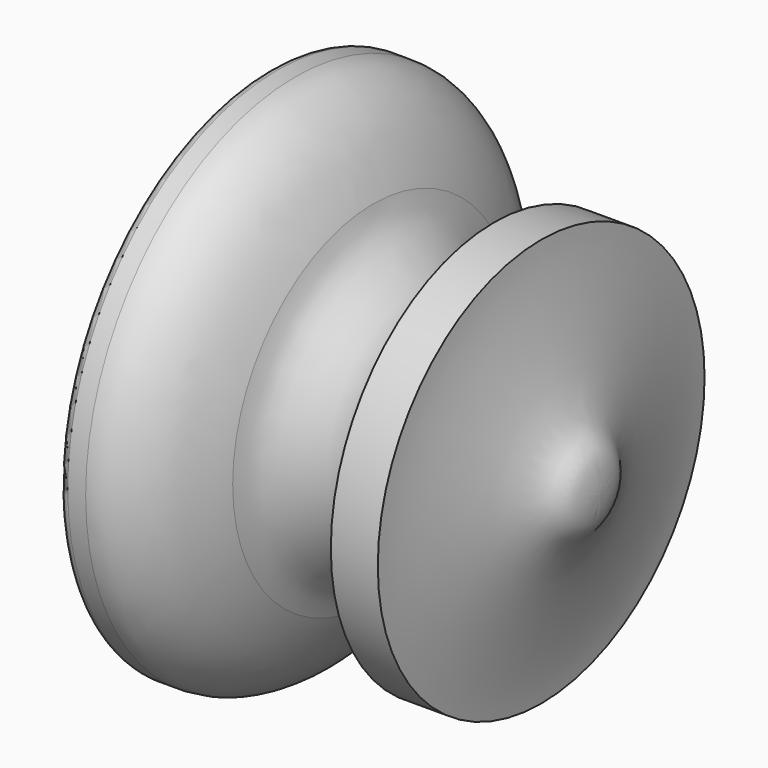
from build123d import *

# Parameters (mm, degrees)
F4_R     = 2.1
F5_DEPTH = 3.5
F6_R     = 0.2
F7_R     = 0.2
F8_R     = 0.2


# Not quite as in the source:
# - ends of sketch curves that miss each other by under 0.0002 mm in the source are joined


with BuildPart() as f2:
    # F1 (on Front) → F2 (revolve)
    with BuildSketch(Plane.XZ):
        with BuildLine():
            Line((45.5202093899, 16.5688355967), (45.5202093899, 14.5688355967))
            add(Edge.make_bspline(
                [(45.5202093899, 14.5688355967), (47.0030293557, 15.1324356496), (50.4613529685, 15.2383481596), (49.5200126524, 9.8090960667), (50.7772336715, 7.0866265215), (51.3850711286, 5.2699102089)],
                knots=[0, 0, 0, 0, 0.3141459464, 0.6391881019, 1, 1, 1, 1], degree=3))
            add(Edge.make_bspline(
                [(51.3850711286, 5.2699102089), (51.9194927912, 3.4284537262), (53.407216137, -1.4620910675), (55.7074866053, -3.3279656709), (55.9983577552, -5.3318521758), (56.1404339969, -6.0311644033)],
                knots=[0, 0, 0, 0, 0.44288519, 0.7345759766, 1, 1, 1, 1], degree=3))
            Line((56.1404339969, -6.0311644033), (57.2202093899, -6.0311644033))
            add(Edge.make_bspline(
                [(50.7202093899, 16.5688355967), (50.8358756015, 14.4597607889), (51.6084715421, 10.0247948502), (52.6677632468, 5.3943286242), (54.7601573389, -1.6439715105), (57.2202093899, -2.029285999), (57.2202093899, -6.0311644033)],
                knots=[0, 0, 0, 0, 0.2620379435, 0.4951606169, 0.7502828141, 1, 1, 1, 1], degree=3))
            Line((50.7202093899, 16.5688355967), (45.5202093899, 16.5688355967))
        make_face()
    revolve(axis=Axis((51.3702093899, 0, -6.0311644033), (-1, 0, 0)))

    # F8
    f8_edges = [f2.edges().sort_by_distance(p)[0] for p in [
        (45.520209, 0, -26.631164),
    ]]
    fillet(f8_edges, radius=F8_R)


with BuildPart() as f3:
    # F0 (on Front) → F3 (revolve)
    with BuildSketch(Plane.XZ):
        with BuildLine():
            Line((36.0301565851, -3.3148658602), (40.5297849349, -3.3148658602))
            Line((40.5297849349, -3.3148658602), (40.5297849349, -2.8144942175))
            ThreePointArc((40.5297849349, -2.8144942175), (40.3834471793, -2.4612036233), (40.0301565851, -2.3148658677))
            Line((40.0301565851, -2.3148658677), (38.2797849349, -2.3148658677))
            Line((38.2797849349, -2.3148658677), (38.2797849349, -1.3148658677))
            Line((38.2797849349, -1.3148658677), (37.8301565851, -1.3148658677))
            ThreePointArc((37.8301565851, -1.3148658677), (37.4763403981, -1.1683104045), (37.3297849349, -0.8144942175))
            Line((37.3297849349, -0.8144942175), (37.3297849349, 0.7809131756))
            ThreePointArc((37.3297849349, 0.7809131756), (37.4742543893, 1.1318977259), (37.8239406894, 1.2794818352))
            Line((37.8239406894, 1.2794818352), (38.4596976111, 1.2851341398))
            Line((38.4596976111, 1.2851341398), (38.4596976111, 1.5851341398))
            Line((38.4596976111, 1.5851341398), (37.2597005307, 1.5877812608))
            Line((37.2597005307, 1.5877812608), (37.2597005307, 4.2877812608))
            Line((37.2597005307, 4.2877812608), (38.4596976111, 4.2851341398))
            add(Edge.make_bspline(
                [(32.1163717198, 14.0041006522), (32.5276845382, 11.6390519459), (35.0915915632, 9.2569192194), (38.4596976111, 6.1171249245), (38.4596976111, 4.2851341398)],
                knots=[0, 0, 0, 0, 0.5043739502, 1, 1, 1, 1], degree=3))
            add(Edge.make_bspline(
                [(23.5099623779, 23.5849531425), (25.0102331097, 23.5849531425), (28.5668995583, 21.3667561799), (30.5941764358, 17.8681345529), (32.1163717198, 14.0041006522)],
                knots=[0, 0, 0, 0, 0.4258635783, 1, 1, 1, 1], degree=3))
            Line((23.5099623779, 23.5849531425), (21.5242667176, 23.5849531425))
            ThreePointArc((21.5242667176, 23.5849531425), (20.8175904861, 23.2915789108), (20.5264681652, 22.5839720071))
            Line((20.5264681652, 22.5839720071), (20.5423877116, 17.5849531425))
            Line((20.5423877116, 17.5849531425), (22.0423801057, 17.5897299195))
            Line((22.0423801057, 17.5897299195), (22.0423801057, 19.9897299195))
            ThreePointArc((22.0423801057, 19.9897299195), (22.3352733245, 20.6968367007), (23.0423801057, 20.9897299195))
            Line((23.0423801057, 20.9897299195), (24.5423801057, 20.9897299195))
            ThreePointArc((24.5423801057, 20.9897299195), (25.2494868869, 20.6968367007), (25.5423801057, 19.9897299195))
            Line((25.5423801057, 19.9897299195), (25.5423801057, 17.5849531425))
            Line((25.5423801057, 17.5849531425), (25.9363012909, 17.5849531425))
            ThreePointArc((25.9363012909, 17.5849531425), (26.196917794, 17.5111367429), (26.3801148345, 17.311615649))
            Line((26.3801148345, 17.311615649), (32.2518409864, 5.6590504444))
            ThreePointArc((32.2518409864, 5.6590504444), (32.6204651827, 5.2575794233), (33.144870756, 5.1090480338))
            Line((33.144870756, 5.1090480338), (33.5281772316, 5.1090480338))
            ThreePointArc((33.5281772316, 5.1090480338), (34.2352840127, 4.816154815), (34.5281772316, 4.1090480338))
            Line((34.5281772316, 4.1090480338), (34.5281772316, 1.903881737))
            ThreePointArc((34.5281772316, 1.903881737), (34.2355702979, 1.1970613569), (33.5289871321, 0.903882065))
            Line((33.5289871321, 0.903882065), (33.5281772316, 0.903881737))
            ThreePointArc((33.5281772316, 0.903881737), (32.8215940661, 0.6107021171), (32.5289871324, -0.096118263))
            Line((32.5289871324, -0.096118263), (32.5289871324, -0.5692796412))
            Line((32.5289871324, -0.5692796412), (32.5289871324, -0.7692796412))
            Line((32.5289871324, -0.7692796412), (32.5289871324, -3.3148658602))
            Line((32.5289871324, -3.3148658602), (36.0301565851, -3.3148658602))
        make_face()
    revolve(axis=Axis((30.5297849349, 0, -5.4148658602), (-1, 0, 0)))

    # F4 (on face) → F5 (cut)
    with BuildSketch(Plane(origin=(32.5289871324, 0, 0), x_dir=(0, -1, 0), z_dir=(-1, 0, 0))):
        Polygon((-2.1939310229, -9.2148658602), (2.1939310229, -9.2148658602), (4.3878620458, -5.4148658602), (2.1939310229, -1.6148658602), (-2.1939310229, -1.6148658602), (-4.3878620458, -5.4148658602), align=None)
        with Locations((0, -5.4148658602)):
            Circle(F4_R, mode=Mode.SUBTRACT)
    extrude(amount=-F5_DEPTH, mode=Mode.SUBTRACT)

    # F6
    f6_edges = [f3.edges().sort_by_distance(p)[0] for p in [
        (36.028987, 0, -9.214866),
        (36.028987, -3.290897, -7.314866),
        (36.028987, -3.290897, -3.514866),
        (36.028987, 0, -1.614866),
        (36.028987, 3.290897, -3.514866),
        (36.028987, 3.290897, -7.314866),
        (36.028987, 0, -7.514866),
    ]]
    fillet(f6_edges, radius=F6_R)

    # F7
    f7_edges = [f3.edges().sort_by_distance(p)[0] for p in [
        (32.528987, 0, -10.733613),
        (32.528987, 0, -9.214866),
        (32.528987, -3.290897, -7.314866),
        (32.528987, -3.290897, -3.514866),
        (32.528987, 0, -1.614866),
        (32.528987, 3.290897, -3.514866),
        (32.528987, 3.290897, -7.314866),
    ]]
    fillet(f7_edges, radius=F7_R)


solid = Compound([f2.part, f3.part])
